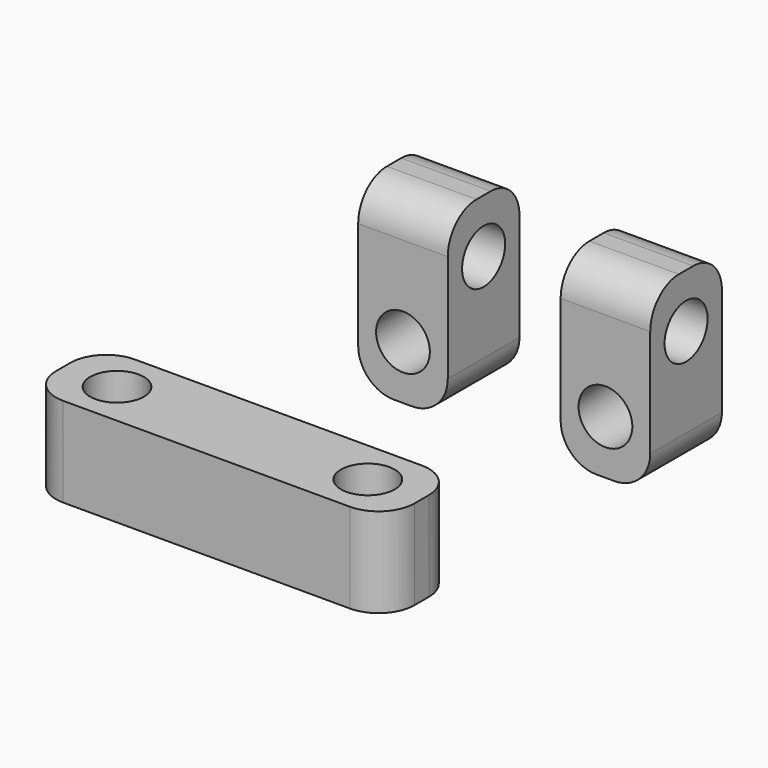
from build123d import *

# Parameters (mm, degrees)
F0_R     = 1.5
F1_DEPTH = 5
F2_W     = 5
F2_H     = 5
F3_DEPTH = 10
F5_R     = 1.5
F6_DEPTH = 25
F4_R     = 1.5
F7_DEPTH = 25
F8_R     = 2


with BuildPart() as f1:
    # F0 (on Top) → F1 (new body)
    with BuildSketch(Plane.XY):
        with BuildLine():
            Line((18, 0), (2, 0))
            ThreePointArc((2, 0), (0.5857864376, -0.5857864376), (0, -2))
            Line((0, -2), (0, -3))
            ThreePointArc((0, -3), (0.5857864376, -4.4142135624), (2, -5))
            Line((2, -5), (18, -5))
            ThreePointArc((18, -5), (19.4142135624, -4.4142135624), (20, -3))
            Line((20, -3), (20, -2))
            ThreePointArc((20, -2), (19.4142135624, -0.5857864376), (18, 0))
        make_face()
        with Locations((3, -2.5)):
            Circle(F0_R, mode=Mode.SUBTRACT)
        with Locations((17, -2.5)):
            Circle(F0_R, mode=Mode.SUBTRACT)
    extrude(amount=F1_DEPTH)


with BuildPart() as f3:
    # F2 (on Top) → F3 (new body)
    with BuildSketch(Plane.XY):
        with Locations((7.687235162, 14.0904001892)):
            Rectangle(F2_W, F2_H)
    extrude(amount=F3_DEPTH)

    # F5 (on face) → F6 (cut)
    with BuildSketch(Plane(origin=(0, 16.5904001892, 0), x_dir=(-1, 0, 0), z_dir=(0, 1, 0))):
        with Locations((-7.687235162, 3)):
            Circle(F5_R)
    extrude(amount=-F6_DEPTH, mode=Mode.SUBTRACT)

    # F4 (on face) → F7 (cut)
    with BuildSketch(Plane(origin=(5.187235162, 0, 0), x_dir=(0, -1, 0), z_dir=(-1, 0, 0))):
        with Locations((-14.0904001892, 7)):
            Circle(F4_R)
    extrude(amount=-F7_DEPTH, mode=Mode.SUBTRACT)

    # F8
    f8_edges = [f3.edges().sort_by_distance(p)[0] for p in [
        (7.687235, 16.5904, 10),
        (7.687235, 11.5904, 10),
        (5.187235, 14.0904, 0),
        (10.187235, 14.0904, 0),
    ]]
    fillet(f8_edges, radius=F8_R)


with BuildPart() as f9_1:
    # F9: copy of F3
    add(f3.part.moved(Location((11.3, 0, 0))))


solid = Compound([f1.part, f3.part, f9_1.part])
